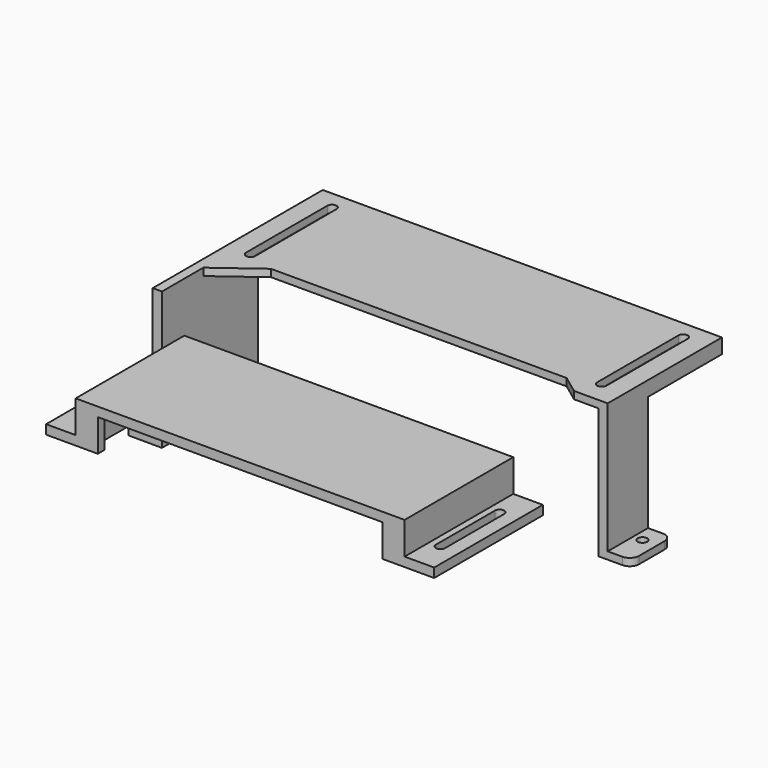
from build123d import *

# Parameters (mm, degrees)
F1_DEPTH  = 65
F2_W      = 160
F2_H      = 45
F3_DEPTH  = 4
F4_W      = 5
F4_H      = 4
F5_DEPTH  = 50
F6_W      = 37.7336093783
F6_H      = 70.5
F6_H_2    = 4.8720824718
F7_DEPTH  = 25
F8_R      = 2.6
F9_DEPTH  = 25
F10_R     = 5
F12_DEPTH = 25
F13_W     = 210
F13_H     = 73.5
F13_W_2   = 185
F13_H_2   = 40
F14_DEPTH = 5
F15_W     = 178
F15_H     = 73.5
F16_DEPTH = 17.5
F17_W     = 165.2
F17_H     = 65.7
F18_DEPTH = 17.5
F19_W     = 154
F19_H     = 17.5
F20_DEPTH = 25
F21_W     = 82.6
F21_H     = 17.5
F22_DEPTH = 25


# Not quite as in the source:
# - a feature names something its author has since deleted; it is built from what else it names


with BuildPart() as f1:
    # F0 (on Front) → F1 (new body)
    with BuildSketch(Plane.XZ):
        Polygon((108, -32.5), (108, 38), (-108, 38), (-108, -32.5), (-120.9999257403, -32.4482956199), (-120.9999257403, -36.4482956199), (-103, -36.5), (-103, 34), (0, 34), (103, 34), (103, -36.5), (120.9999257403, -36.4482956199), (120.9999257403, -32.4482956199), align=None)
    extrude(amount=F1_DEPTH)

    # F2 (on face) → F3 (cut, through all)
    with BuildSketch(Plane.XY.offset(38)):
        with Locations((0, -42.5)):
            Rectangle(F2_W, F2_H)
        Polygon((80, -20), (80, -65), (107, -65), (107, -40), align=None)
        Polygon((-103, -65), (-80, -65), (-80, -20), (-103, -37.037037037), align=None)
    extrude(amount=-F3_DEPTH, mode=Mode.SUBTRACT)

    # F4 (on face) → F5 (join)
    with BuildSketch(Plane(origin=(0, 0, 0), x_dir=(-1, 0, 0), z_dir=(0, 1, 0))):
        Polygon((103, 38), (-108, 38), (-108, 34), (-103, 34), (103, 34), align=None)
        with Locations((-105.5, 32)):
            Rectangle(F4_W, F4_H)
        Polygon((108, 38), (103, 38), (103, 34), (103, 30), (108, 30), (108, 34), align=None)
    extrude(amount=F5_DEPTH)

    # F6 (on face) → F7 (cut, symmetric)
    with BuildSketch(Plane.YZ.offset(108)):
        with Locations((-46.1331953108, 2.75)):
            Rectangle(F6_W, F6_H)
        with Locations((-46.1331953108, -34.9360412359)):
            Rectangle(F6_W, F6_H_2)
    extrude(amount=F7_DEPTH, both=True, mode=Mode.SUBTRACT)

    # F8 (on face) → F9 (cut)
    with BuildSketch(Plane(origin=(-0.1056944195, 0, -36.7955615686), x_dir=(0.9999958745, 0, -0.0028724656), z_dir=(-0.0028724656, 0, -0.9999958745))):
        with BuildLine():
            ThreePointArc((-112.8947300766, 12.6), (-114.7332077077, 8.1615223689), (-110.2947300766, 10))
            ThreePointArc((-110.2947300766, 10), (-111.0562524455, 11.8384776311), (-112.8947300766, 12.6))
        make_face()
        with BuildLine():
            ThreePointArc((-110.2947300766, 55), (-114.7332077077, 56.8384776311), (-112.8947300766, 52.4))
            ThreePointArc((-112.8947300766, 52.4), (-111.0562524455, 53.1615223689), (-110.2947300766, 55))
        make_face()
        with Locations((113.1061197876, 55)):
            Circle(F8_R)
        with Locations((113.1061197876, 10)):
            Circle(F8_R)
    extrude(amount=-F9_DEPTH, mode=Mode.SUBTRACT)

    # F10
    f10_edges = [f1.edges().sort_by_distance(p)[0] for p in [
        (120.999926, 0, -34.448296),
        (120.999926, -27.266391, -34.448296),
    ]]
    fillet(f10_edges, radius=F10_R)

    # F11 (on face) → F12 (cut)
    with BuildSketch(Plane.XY.offset(38)):
        with BuildLine():
            Line((-95, 40), (-92.5, 40))
            ThreePointArc((-92.5, 40), (-95, 42.5), (-97.5, 40))
            ThreePointArc((-97.5, 40), (-96.767766953, 38.232233047), (-95, 37.5))
            Line((-95, 37.5), (-95, 40))
        make_face()
        with BuildLine():
            ThreePointArc((-95, 37.5), (-93.232233047, 38.232233047), (-92.5, 40))
            Line((-92.5, 40), (-95, 40))
            Line((-95, 40), (-95, 37.5))
        make_face()
        with BuildLine():
            Line((-92.5, 0), (-95, 0))
            Line((-95, 0), (-95, 2.5))
            ThreePointArc((-95, 2.5), (-96.767766953, 1.767766953), (-97.5, 0))
            ThreePointArc((-97.5, 0), (-95, -2.5), (-92.5, 0))
        make_face()
        with BuildLine():
            Line((-95, 2.5), (-95, 0))
            Line((-95, 0), (-92.5, 0))
            ThreePointArc((-92.5, 0), (-93.232233047, 1.767766953), (-95, 2.5))
        make_face()
        with BuildLine():
            Line((95, 0), (92.5, 0))
            ThreePointArc((92.5, 0), (93.232233047, -1.767766953), (95, -2.5))
            Line((95, -2.5), (95, 0))
        make_face()
        with BuildLine():
            ThreePointArc((95, 2.5), (93.232233047, 1.767766953), (92.5, 0))
            Line((92.5, 0), (95, 0))
            Line((95, 0), (95, 2.5))
        make_face()
        with BuildLine():
            ThreePointArc((97.5, 40), (95, 42.5), (92.5, 40))
            Line((92.5, 40), (95, 40))
            Line((95, 40), (95, 37.5))
            ThreePointArc((95, 37.5), (96.767766953, 38.232233047), (97.5, 40))
        make_face()
        with BuildLine():
            Line((95, 40), (92.5, 40))
            ThreePointArc((92.5, 40), (93.232233047, 38.232233047), (95, 37.5))
            Line((95, 37.5), (95, 40))
        make_face()
        with BuildLine():
            Line((95, 37.5), (95, 2.5))
            ThreePointArc((95, 2.5), (96.767766953, 1.767766953), (97.5, 0))
            Line((97.5, 0), (97.5, 40))
            ThreePointArc((97.5, 40), (96.767766953, 38.232233047), (95, 37.5))
        make_face()
        with BuildLine():
            Line((95, 2.5), (95, 0))
            Line((95, 0), (95, -2.5))
            ThreePointArc((95, -2.5), (96.767766953, -1.767766953), (97.5, 0))
            ThreePointArc((97.5, 0), (96.767766953, 1.767766953), (95, 2.5))
        make_face()
        with BuildLine():
            ThreePointArc((97.5, 0), (96.767766953, -1.767766953), (95, -2.5))
            Line((95, -2.5), (95, -12.5))
            ThreePointArc((95, -12.5), (96.767766953, -13.232233047), (97.5, -15))
            Line((97.5, -15), (97.5, 0))
        make_face()
        with BuildLine():
            ThreePointArc((95, -12.5), (93.232233047, -13.232233047), (92.5, -15))
            ThreePointArc((92.5, -15), (95, -17.5), (97.5, -15))
            ThreePointArc((97.5, -15), (96.767766953, -13.232233047), (95, -12.5))
        make_face()
        with BuildLine():
            Line((92.5, 40), (92.5, 0))
            ThreePointArc((92.5, 0), (93.232233047, 1.767766953), (95, 2.5))
            Line((95, 2.5), (95, 37.5))
            ThreePointArc((95, 37.5), (93.232233047, 38.232233047), (92.5, 40))
        make_face()
        with BuildLine():
            ThreePointArc((95, -2.5), (93.232233047, -1.767766953), (92.5, 0))
            Line((92.5, 0), (92.5, -15))
            ThreePointArc((92.5, -15), (93.232233047, -13.232233047), (95, -12.5))
            Line((95, -12.5), (95, -2.5))
        make_face()
        with BuildLine():
            ThreePointArc((-95, 2.5), (-93.232233047, 1.767766953), (-92.5, 0))
            Line((-92.5, 0), (-92.5, 40))
            ThreePointArc((-92.5, 40), (-93.232233047, 38.232233047), (-95, 37.5))
            Line((-95, 37.5), (-95, 2.5))
        make_face()
        with BuildLine():
            ThreePointArc((-97.5, 0), (-96.767766953, 1.767766953), (-95, 2.5))
            Line((-95, 2.5), (-95, 37.5))
            ThreePointArc((-95, 37.5), (-96.767766953, 38.232233047), (-97.5, 40))
            Line((-97.5, 40), (-97.5, 0))
        make_face()
        with BuildLine():
            ThreePointArc((-97.5, -15), (-95, -17.5), (-92.5, -15))
            ThreePointArc((-92.5, -15), (-95, -12.5), (-97.5, -15))
        make_face()
        with BuildLine():
            Line((-92.5, -15), (-92.5, 0))
            ThreePointArc((-92.5, 0), (-95, -2.5), (-97.5, 0))
            Line((-97.5, 0), (-97.5, -15))
            ThreePointArc((-97.5, -15), (-95, -12.5), (-92.5, -15))
        make_face()
    extrude(amount=-F12_DEPTH, mode=Mode.SUBTRACT)


with BuildPart() as f14:
    # F13 (on Top) → F14 (new body)
    with BuildSketch(Plane.XY):
        with Locations((0, -104.1353195906)):
            Rectangle(F13_W, F13_H)
        with BuildLine():
            ThreePointArc((97.5, -124.1353195906), (95, -126.6353195906), (92.5, -124.1353195906))
            Line((92.5, -124.1353195906), (-92.5, -124.1353195906))
            ThreePointArc((-92.5, -124.1353195906), (-95, -126.6353195906), (-97.5, -124.1353195906))
            Line((-97.5, -124.1353195906), (-97.5, -84.1353195906))
            ThreePointArc((-97.5, -84.1353195906), (-95, -81.6353195906), (-92.5, -84.1353195906))
            Line((-92.5, -84.1353195906), (92.5, -84.1353195906))
            ThreePointArc((92.5, -84.1353195906), (95, -81.6353195906), (97.5, -84.1353195906))
            Line((97.5, -84.1353195906), (97.5, -124.1353195906))
        make_face(mode=Mode.SUBTRACT)
        with Locations((0, -104.1353195906)):
            Rectangle(F13_W_2, F13_H_2)
    extrude(amount=F14_DEPTH)

    # F15 (on face) → F16 (join)
    with BuildSketch(Plane.XY.offset(5)):
        with Locations((0, -104.1353195906)):
            Rectangle(F15_W, F15_H)
    extrude(amount=F16_DEPTH)

    # F17 (on face) → F18 (cut)
    with BuildSketch(Plane(origin=(0, 0, 0), x_dir=(1, 0, 0), z_dir=(0, 0, -1))):
        with Locations((0, 103.6443784833)):
            Rectangle(F17_W, F17_H)
    extrude(amount=-F18_DEPTH, mode=Mode.SUBTRACT)

    # F19 (on face) → F20 (cut)
    with BuildSketch(Plane.XZ.offset(140.8853195906)):
        with Locations((0, 8.75)):
            Rectangle(F19_W, F19_H)
    extrude(amount=-F20_DEPTH, mode=Mode.SUBTRACT)

    # F21 (on face) → F22 (cut)
    with BuildSketch(Plane.XZ.offset(70.7943784833)):
        with Locations((41.3, 8.75)):
            Rectangle(F21_W, F21_H)
    extrude(amount=-F22_DEPTH, mode=Mode.SUBTRACT)


solid = Compound([f1.part, f14.part])
